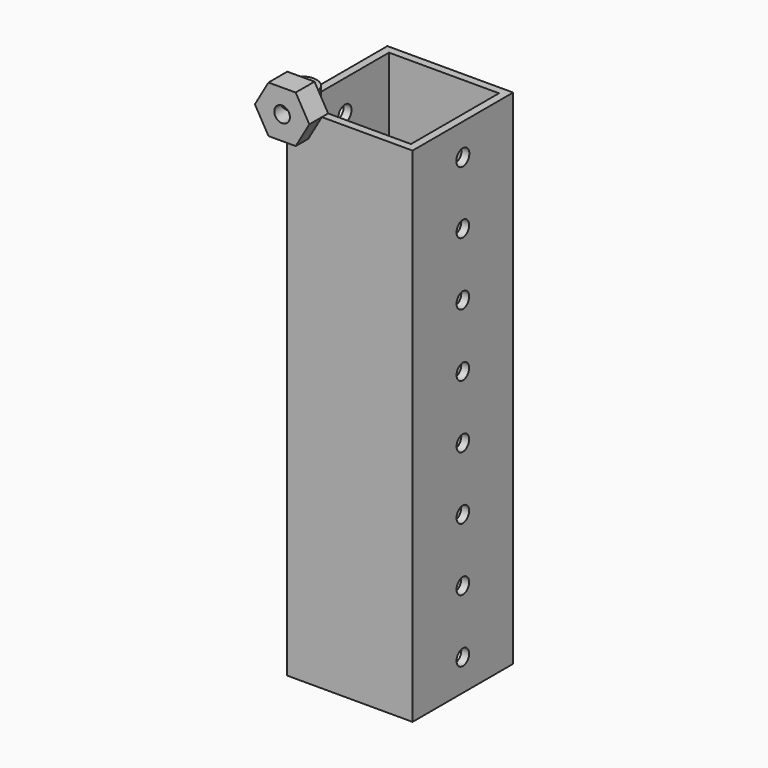
from build123d import *

# Parameters (mm, degrees)
F2_DEPTH  = 4.7625
F1_R      = 1.58301057
F3_DEPTH  = 4.7625
F4_R      = 3.175
F5_DEPTH  = 3.175
F6_R      = 1.5875
F7_DEPTH  = 34.925
F9_DEPTH  = 3.1496
F11_W     = 25.4
F11_H     = 25.4
F12_DEPTH = 101.6
F10_W     = 22.225
F10_H     = 22.225
F13_DEPTH = 101.6
F14_R     = 1.6482662837
F22_DEPTH = 25.4
F15_R     = 1.5875
F23_DEPTH = 25.4
F21_R     = 1.5875
F24_DEPTH = 25.4
F20_R     = 1.5875
F25_DEPTH = 25.4
F19_R     = 1.5875
F26_DEPTH = 25.4
F18_R     = 1.5875
F27_DEPTH = 25.4
F17_R     = 1.5875
F28_DEPTH = 25.4
F16_R     = 1.5875
F29_DEPTH = 25.4


with BuildPart() as f2:
    # F0 (on Front) → F2 (new body)
    with BuildSketch(Plane.XZ):
        Polygon((2.7564916063, -4.7585388291), (5.499261314, 0.0079223418), (2.7427697078, 4.7664611709), (-2.7564916063, 4.7585388291), (-5.499261314, -0.0079223418), (-2.7427697078, -4.7664611709), align=None)
    extrude(amount=F2_DEPTH)

    # F1 (on face) → F3 (cut)
    with BuildSketch(Plane.XZ):
        Circle(F1_R)
    extrude(amount=F3_DEPTH, mode=Mode.SUBTRACT)


with BuildPart() as f5:
    # F4 (on Top) → F5 (new body)
    with BuildSketch(Plane.XY):
        Circle(F4_R)
    extrude(amount=F5_DEPTH)

    # F6 (on face) → F7 (join)
    with BuildSketch(Plane(origin=(0, 0, 0), x_dir=(1, 0, 0), z_dir=(0, 0, -1))):
        Circle(F6_R)
    extrude(amount=F7_DEPTH)

    # F8 (on face) → F9 (cut)
    with BuildSketch(Plane.XY.offset(3.175)):
        Polygon((-1.5875, 0.9165435523), (-1.5875, -0.9165435523), (0, -1.8330871047), (1.5875, -0.9165435523), (1.5875, 0.9165435523), (0, 1.8330871047), align=None)
    extrude(amount=-F9_DEPTH, mode=Mode.SUBTRACT)


with BuildPart() as f12:
    # F11 (on Top) → F12 (new body)
    with BuildSketch(Plane.XY):
        with Locations((11.1125, 11.1125)):
            Rectangle(F11_W, F11_H)
    extrude(amount=-F12_DEPTH)

    # F10 (on Top) → F13 (cut)
    with BuildSketch(Plane.XY):
        with Locations((11.1125, 11.1125)):
            Rectangle(F10_W, F10_H)
    extrude(amount=-F13_DEPTH, mode=Mode.SUBTRACT)

    # F14 (on face) → F22 (cut)
    with BuildSketch(Plane.YZ.offset(23.8125)):
        with Locations((11.1125, -6.35)):
            Circle(F14_R)
    extrude(amount=-F22_DEPTH, mode=Mode.SUBTRACT)

    # F15 (on face) → F23 (cut)
    with BuildSketch(Plane.YZ.offset(23.8125)):
        with Locations((11.1125, -19.05)):
            Circle(F15_R)
    extrude(amount=-F23_DEPTH, mode=Mode.SUBTRACT)

    # F21 (on face) → F24 (cut)
    with BuildSketch(Plane.YZ.offset(23.8125)):
        with Locations((11.1125, -95.25)):
            Circle(F21_R)
    extrude(amount=-F24_DEPTH, mode=Mode.SUBTRACT)

    # F20 (on face) → F25 (cut)
    with BuildSketch(Plane.YZ.offset(23.8125)):
        with Locations((11.1125, -82.55)):
            Circle(F20_R)
    extrude(amount=-F25_DEPTH, mode=Mode.SUBTRACT)

    # F19 (on face) → F26 (cut)
    with BuildSketch(Plane.YZ.offset(23.8125)):
        with Locations((11.1125, -69.85)):
            Circle(F19_R)
    extrude(amount=-F26_DEPTH, mode=Mode.SUBTRACT)

    # F18 (on face) → F27 (cut)
    with BuildSketch(Plane.YZ.offset(23.8125)):
        with Locations((11.1125, -57.15)):
            Circle(F18_R)
    extrude(amount=-F27_DEPTH, mode=Mode.SUBTRACT)

    # F17 (on face) → F28 (cut)
    with BuildSketch(Plane.YZ.offset(23.8125)):
        with Locations((11.1125, -44.45)):
            Circle(F17_R)
    extrude(amount=-F28_DEPTH, mode=Mode.SUBTRACT)

    # F16 (on face) → F29 (cut)
    with BuildSketch(Plane.YZ.offset(23.8125)):
        with Locations((11.1125, -31.75)):
            Circle(F16_R)
    extrude(amount=-F29_DEPTH, mode=Mode.SUBTRACT)


solid = Compound([f2.part, f5.part, f12.part])
